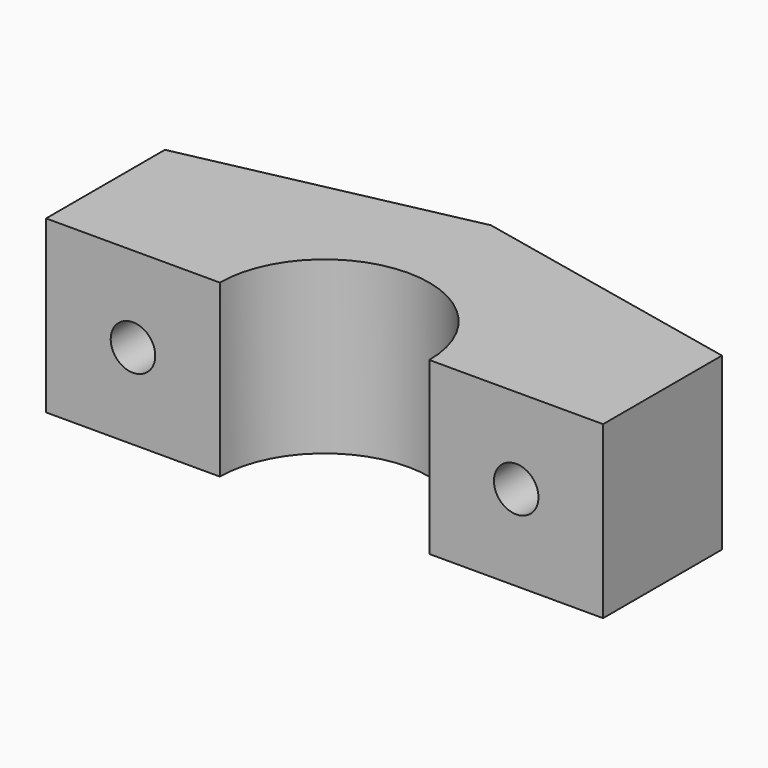
from build123d import *

# Parameters (mm, degrees)
F1_DEPTH  = 23
F4_D      = 6
F5_D      = 6
F6_W      = 75
F6_H      = 5.3172297776
F7_DEPTH  = 8
F8_SIZE2  = 37.5
F8_SIZE   = 8
F9_SIZE2  = 37.5
F9_SIZE   = 8
F10_SIZE2 = 37.49999
F10_SIZE  = 7.99999
F11_SIZE2 = 37.49999
F11_SIZE  = 7.99999
F12_R     = 8.65
F13_DEPTH = 4


# Not quite as in the source:
# - a fillet or chamfer is up to 0.001 mm smaller than in the source, because OpenCascade refuses the exact size


with BuildPart() as f1:
    # F0 (on Top) → F1 (new body)
    with BuildSketch(Plane.XY):
        with BuildLine():
            Line((37.5, 20), (-37.5, 20))
            Line((-37.5, 20), (-37.5, 0))
            Line((-37.5, 0), (-14.1, 0))
            ThreePointArc((-14.1, 0), (0, 14.1), (14.1, 0))
            Line((14.1, 0), (37.5, 0))
            Line((37.5, 0), (37.5, 20))
        make_face()
    extrude(amount=F1_DEPTH)

    # F4 (through all)
    with Locations(Plane.XZ):
        with Locations((-25.8, 11.5)):
            Hole(F4_D / 2)

    # F5 (through all)
    with Locations(Plane.XZ):
        with Locations((25.8, 11.5)):
            Hole(F5_D / 2)

    # F6 (on face) → F7 (join)
    with BuildSketch(Plane(origin=(0, 20, 0), x_dir=(-1, 0, 0), z_dir=(0, 1, 0))):
        with Locations((0, 20.3413851112)):
            Rectangle(F6_W, F6_H)
        with Locations((0, 2.6586148888)):
            Rectangle(F6_W, F6_H)
    extrude(amount=F7_DEPTH)

    # F8
    f8_edges = [f1.edges().sort_by_distance(p)[0] for p in [
        (37.5, 28, 2.658615),
    ]]
    f8_side = f1.faces().sort_by_distance((37.5, 12.185127, 11.5))[0]
    chamfer(f8_edges, length=F8_SIZE, length2=F8_SIZE2, reference=f8_side)

    # F9
    f9_edges = [f1.edges().sort_by_distance(p)[0] for p in [
        (37.5, 28, 20.341385),
    ]]
    f9_side = f1.faces().sort_by_distance((37.5, 11.185045, 12.248388))[0]
    chamfer(f9_edges, length=F9_SIZE, length2=F9_SIZE2, reference=f9_side)

    # F10 (size 8 and 37.5 in the source; OpenCascade refuses exactly that, so slightly less here)
    f10_edges = [f1.edges().sort_by_distance(p)[0] for p in [
        (-37.5, 28, 20.341385),
    ]]
    f10_side = f1.faces().sort_by_distance((-37.5, 12.185127, 11.5))[0]
    chamfer(f10_edges, length=F10_SIZE, length2=F10_SIZE2, reference=f10_side)

    # F11 (size 8 and 37.5 in the source; OpenCascade refuses exactly that, so slightly less here)
    f11_edges = [f1.edges().sort_by_distance(p)[0] for p in [
        (-37.5, 28, 2.658615),
    ]]
    f11_side = f1.faces().sort_by_distance((-37.5, 11.185046, 10.751613))[0]
    chamfer(f11_edges, length=F11_SIZE, length2=F11_SIZE2, reference=f11_side)

    # F12 (on face) → F13 (cut, symmetric)
    with BuildSketch(Plane(origin=(0, 20, 0), x_dir=(-1, 0, 0), z_dir=(0, 1, 0))):
        with Locations((25.8, 11.5)):
            Circle(F12_R)
        with Locations((-25.8, 11.5)):
            Circle(F12_R)
    extrude(amount=F13_DEPTH, both=True, mode=Mode.SUBTRACT)


solid = f1.part
